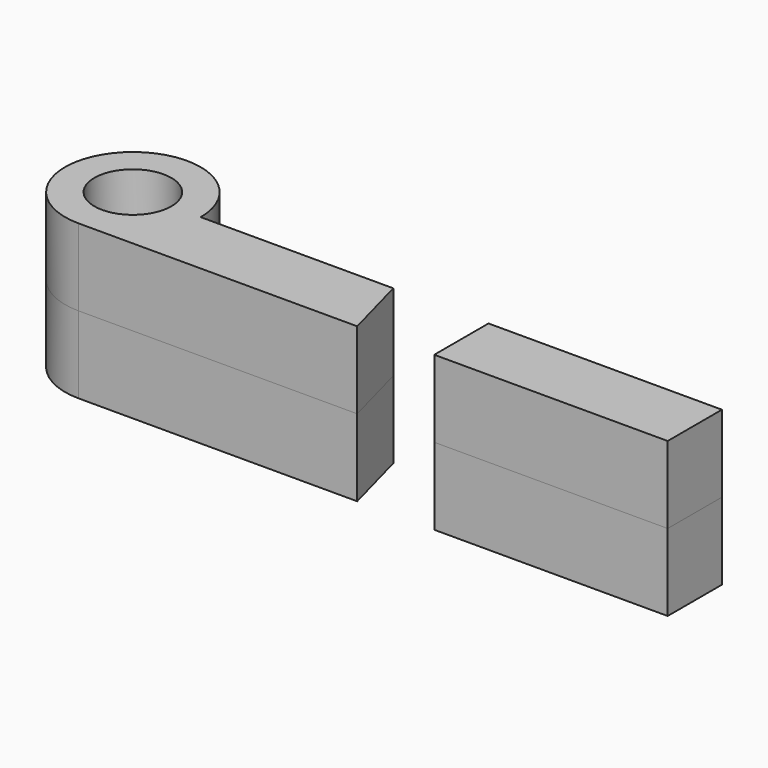
from build123d import *

# Parameters (mm, degrees)
F0_W     = 76.962
F0_H     = 22.352
F1_DEPTH = 25.4
F2_DEPTH = 25.4


with BuildPart() as f1:
    # F0 (on Top) → F1 (new body)
    with BuildSketch(Plane.XY):
        with BuildLine():
            Line((22.352, 0), (12.7, 0))
            ThreePointArc((12.7, 0), (8.9802561211, -8.9802561211), (0, -12.7))
            Line((0, -12.7), (0, -22.352))
            ThreePointArc((0, -22.352), (15.8052507731, -15.8052507731), (22.352, 0))
        make_face()
        with BuildLine():
            ThreePointArc((0, -12.7), (-8.9802561211, 8.9802561211), (12.7, 0))
            Line((12.7, 0), (22.352, 0))
            ThreePointArc((22.352, 0), (-15.8052507731, 15.8052507731), (0, -22.352))
            Line((0, -22.352), (0, -12.7))
        make_face()
        with BuildLine():
            Line((85.852, 0), (22.352, 0))
            ThreePointArc((22.352, 0), (15.8052507731, -15.8052507731), (0, -22.352))
            Line((0, -22.352), (91.8464, -22.352))
            Line((91.8464, -22.352), (85.852, 0))
        make_face()
        Polygon((117.2464, 0), (85.852, 0), (91.8464, -22.352), (117.2464, -22.352), align=None)
        with Locations((155.7274, -11.176)):
            Rectangle(F0_W, F0_H)
    extrude(amount=F1_DEPTH)

    # F0 (on Top) → F2 (cut)
    with BuildSketch(Plane.XY):
        Polygon((117.2464, 0), (85.852, 0), (91.8464, -22.352), (117.2464, -22.352), align=None)
    extrude(amount=F2_DEPTH, mode=Mode.SUBTRACT)


with BuildPart() as f3_1:
    # F3: instance of F1
    add(f1.part.mirror(Plane.XY))


solid = Compound([f1.part, f3_1.part])
